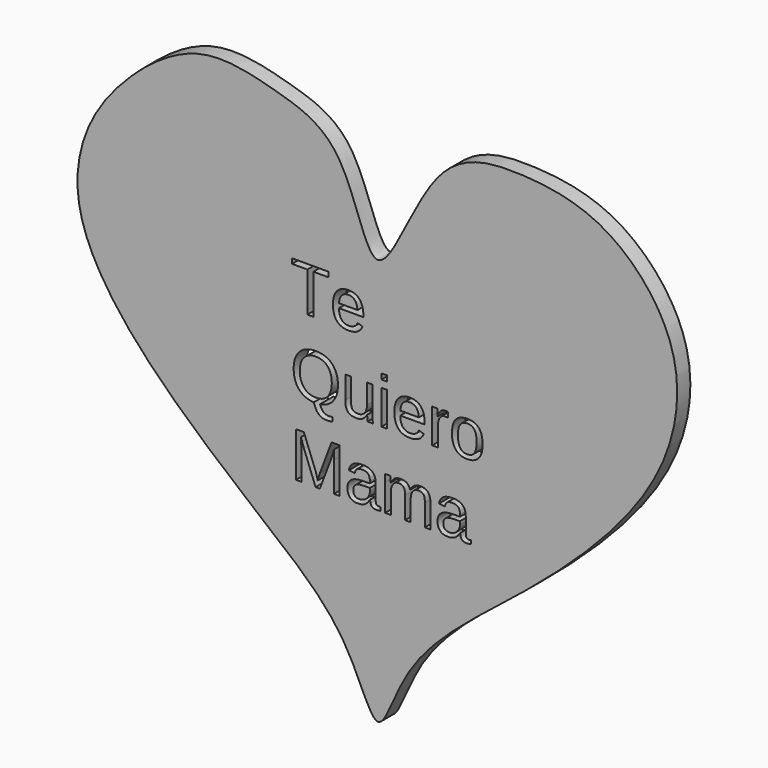
from build123d import *

# Parameters (mm, degrees)
F1_DEPTH     = 3.175
F2_TEXT_SIZE = 12.5236111111
F3_DEPTH     = 3.1760001


# Not quite as in the source:
# - Text() gives the source's letters only with a copy of the font that has no kerning and outlines rounded to 1/6400 em; it was checked with that copy


with BuildPart() as f1:
    # F0 (on Front) → F1 (new body)
    with BuildSketch(Plane.XZ):
        with BuildLine():
            add(Edge.make_bspline(
                [(0, 26.1101331562), (-2.480428239, 26.1504554911), (-5.7992033328, 44.2361885369), (-19.5101796499, 48.4625383962), (-34.8527495659, 52.4583612398), (-49.7802296968, 40.9782528393), (-57.6872285381, 29.0440051631), (-59.0505828839, 13.6933884328), (-46.0347271661, -5.8112311738), (-21.2823757387, -26.0388281085), (-5.6523513067, -38.9164474178), (0.1684201298, -57.9937022552), (5.1680722704, -38.1059242445), (28.172433837, -22.1143774786), (50.1427964885, -1.4392495696), (58.5867815979, 16.3411625194), (57.5605527457, 32.9246476077), (44.3828162364, 47.5902350863), (27.0045990319, 50.3288948933), (10.0057393735, 48.703287246), (2.8360226774, 26.0640302073), (0, 26.1101331562)],
                knots=[0, 0, 0, 0, 0.049665714, 0.0961312181, 0.1431304262, 0.194271395, 0.2403188489, 0.2857254171, 0.343961378, 0.4136873675, 0.4711496011, 0.5135054786, 0.555861357, 0.6227067333, 0.6903804851, 0.7433452178, 0.7913034875, 0.8434741362, 0.8938951971, 0.9432142044, 1, 1, 1, 1], degree=3))
        make_face()
    extrude(amount=F1_DEPTH)

    # F2 (on Front) → F3 (cut, through all)
    with BuildSketch(Plane.XZ):
        with Locations((-16.8628329011, 12.3817092735)):
            Text('Te', F2_TEXT_SIZE, font='Arimo', text_align=(TextAlign.LEFT, TextAlign.BOTTOM))
        with Locations((-16.8628329011, -2.0204435043)):
            Text('Quiero', F2_TEXT_SIZE, font='Arimo', text_align=(TextAlign.LEFT, TextAlign.BOTTOM))
        with Locations((-16.8628329011, -16.4225962821)):
            Text('Mama', F2_TEXT_SIZE, font='Arimo', text_align=(TextAlign.LEFT, TextAlign.BOTTOM))
    extrude(amount=F3_DEPTH, mode=Mode.SUBTRACT)


solid = f1.part
